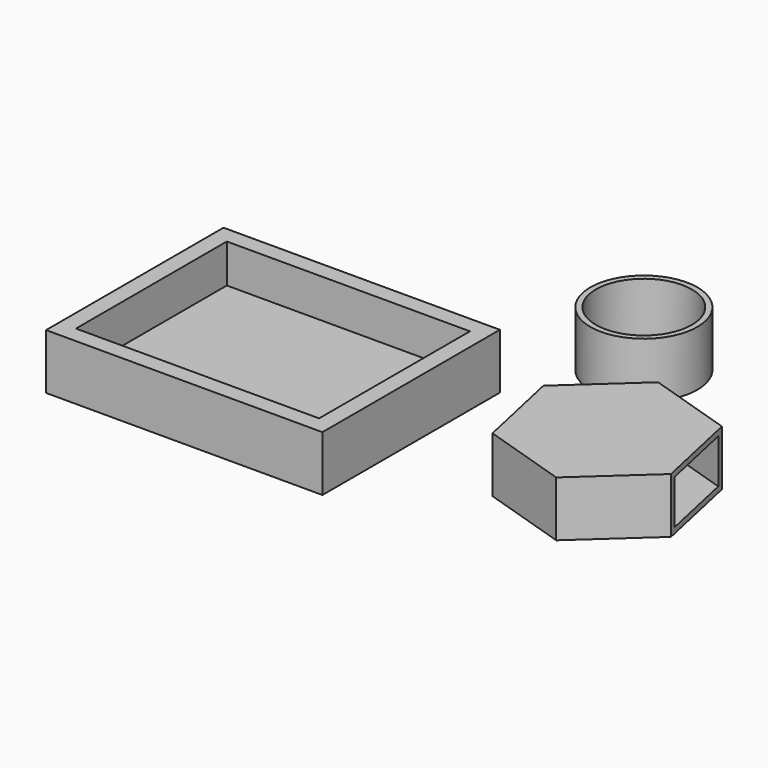
from build123d import *

# Parameters (mm, degrees)
F0_W     = 126.7988150939
F0_H     = 101.7564386129
F1_DEPTH = 25.4
F0_R     = 24.5739182838
F2_T     = -7.62
F3_T     = -2.54
F4_T     = -2.54


# Not quite as in the source:
# - a feature of the source that left no trace in its solid (it failed there, or was rolled back) is left out


with BuildPart() as f1:
    # F0 (on Top) → F1 (new body)
    with BuildSketch(Plane.XY):
        with Locations((-52.4532389827, -50.8782193065)):
            Rectangle(F0_W, F0_H)
    extrude(amount=F1_DEPTH)

    # F2
    f2_openings = [f1.faces().sort_by_distance(p)[0] for p in [
        (-52.453239, -50.878219, 25.4),
    ]]
    offset(amount=F2_T, openings=f2_openings)


with BuildPart() as f1b:
    # F0 (on Top) → F1, piece 2 (new body)
    with BuildSketch(Plane.XY):
        with Locations((40.2616634965, 45.9529422224)):
            Circle(F0_R)
    extrude(amount=F1_DEPTH)

    # F3
    f3_openings = [f1b.faces().sort_by_distance(p)[0] for p in [
        (40.261663, 45.952942, 25.4),
    ]]
    offset(amount=F3_T, openings=f3_openings)


with BuildPart() as f1c:
    # F0 (on Top) → F1, piece 3 (new body)
    with BuildSketch(Plane.XY):
        Polygon((98.3106148388, -76.8574930794), (128.7498819683, -49.104034149), (119.9343150564, -8.866126077), (80.679481015, 3.6183230645), (50.2402138855, -24.1351358659), (59.0557807974, -64.3730439379), align=None)
    extrude(amount=F1_DEPTH)

    # F4
    f4_openings = [f1c.faces().sort_by_distance(p)[0] for p in [
        (124.342099, -28.98508, 12.7),
    ]]
    offset(amount=F4_T, openings=f4_openings)


solid = Compound([f1.part, f1b.part, f1c.part])
